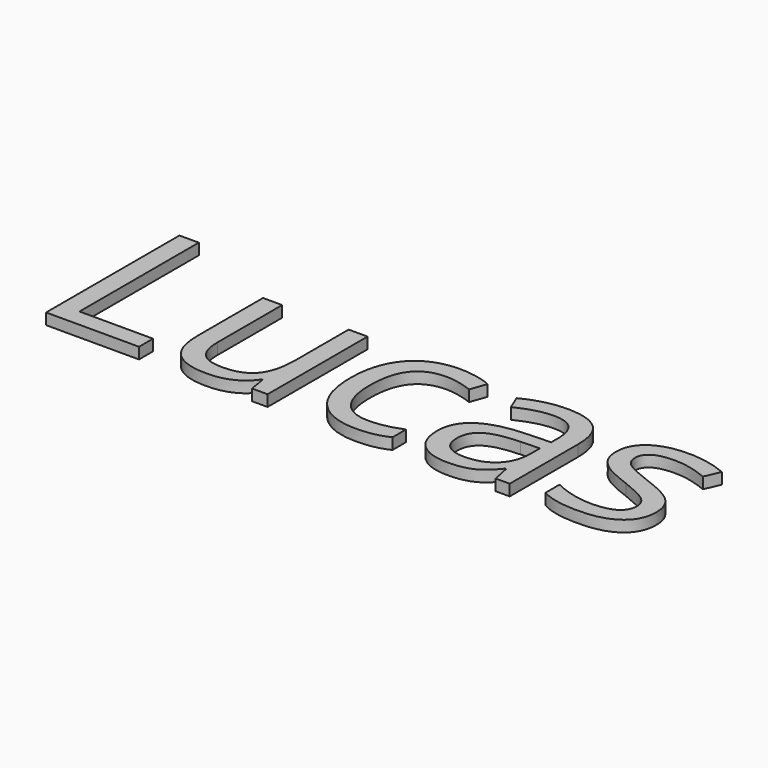
from build123d import *

# Parameters (mm, degrees)
F0_TEXT_SIZE = 20.8333333333
F1_DEPTH     = 1


# Not quite as in the source:
# - Text() gives the source's letters only with a copy of the font that has no kerning and outlines rounded to 1/6400 em; it was checked with that copy


with BuildPart() as f1:
    # F0 (on Top) → F1 (new body)
    with BuildSketch(Plane.XY):
        with Locations((-23.7423306715, 1.2883425345)):
            Text('Lucas', F0_TEXT_SIZE, font='Open Sans', text_align=(TextAlign.LEFT, TextAlign.BOTTOM))
    extrude(amount=F1_DEPTH)


solid = f1.part
